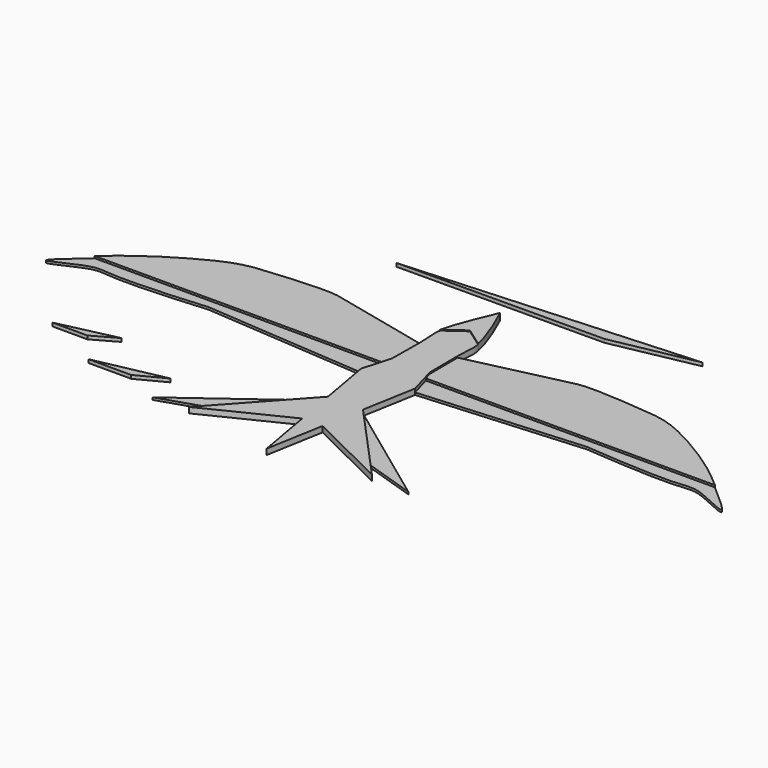
from build123d import *

# Parameters (mm, degrees)
F1_DEPTH = 2
F2_DEPTH = 2.3
F3_DEPTH = 1.5
F4_DEPTH = 0.8
F5_DEPTH = 1.2


# Not quite as in the source:
# - a feature names something its author has since deleted; it is built from what else it names


with BuildPart() as f1:
    # F0 (on Top) → F1 (new body)
    with BuildSketch(Plane.XY):
        with BuildLine():
            Line((-6.6419716499, 2.745028284), (0, 0))
            Line((0, 0), (0, 28.6946911365))
            Line((0, 28.6946911365), (-6.6419716499, 23.9225961235))
            add(Edge.make_bspline(
                [(-6.5175706139, 15.0729201773), (-6.5414876506, 16.2812130784), (-6.6806623081, 20.0881688925), (-7.0635559844, 21.7026716796), (-6.6419716499, 23.9225961235)],
                knots=[0.2785134471, 0.2785134471, 0.2785134471, 0.2785134471, 0.3682433903, 0.5898063865, 0.5898063865, 0.5898063865, 0.5898063865], degree=3))
            add(Edge.make_bspline(
                [(-6.6419716499, 2.745028284), (-6.5251722943, 6.5032297687), (-6.4433343436, 11.3224907311), (-6.5175706139, 15.0729201773)],
                knots=[0, 0, 0, 0, 0.2785134471, 0.2785134471, 0.2785134471, 0.2785134471], degree=3))
        make_face()
        with BuildLine():
            Line((0, 28.6946911365), (0, 0))
            Line((0, 0), (6.6419716499, 2.745028284))
            add(Edge.make_bspline(
                [(6.6419716499, 2.745028284), (6.6625704877, 4.4259580865), (6.6879671442, 8.5489520633), (6.5628964948, 13.2490139748), (6.5686901265, 15.0847156957)],
                knots=[0, 0, 0, 0, 0.2083076988, 0.3619822263, 0.3619822263, 0.3619822263, 0.3619822263], degree=3))
            add(Edge.make_bspline(
                [(6.5686901265, 15.0847156957), (6.5717947616, 16.0684137089), (6.6405692543, 19.2909426976), (7.065262223, 21.4932328604), (6.6419716499, 23.9949107423)],
                knots=[0.3619822263, 0.3619822263, 0.3619822263, 0.3619822263, 0.4443318399, 0.644940685, 0.644940685, 0.644940685, 0.644940685], degree=3))
            Line((6.6419716499, 23.9949107423), (0, 28.6946911365))
        make_face()
        Polygon((9.5007317222, -7.3481148503), (0, -8.0477236517), (0, -38.9328375459), (3.5725845946, -40.6871710497), (6.1658886261, -26.1027980596), align=None)
        Polygon((0, -38.9328375459), (0, -8.0477236517), (-9.5007317222, -7.3481148503), (-6.1658886261, -26.1027980596), (-3.5725845946, -40.6871710497), align=None)
        Polygon((-32.2535888602, -54.7711053479), (-3.5725845946, -40.6871710497), (-6.1658886261, -26.1027980596), (-26.8448407595, -48.8273214495), align=None)
        Polygon((26.8448407595, -48.8273214495), (6.1658886261, -26.1027980596), (3.5725845946, -40.6871710497), (32.2535888602, -54.7711053479), align=None)
        Polygon((0, -8.0477236517), (0, 0), (-7.4194675351, 0), (-9.5007317222, -7.3481148503), align=None)
        Polygon((7.4194675351, 0), (0, 0), (0, -8.0477236517), (9.5007317222, -7.3481148503), align=None)
        Polygon((6.6419716499, 2.745028284), (0, 0), (7.4194675351, 0), align=None)
        Polygon((-7.4194675351, 0), (0, 0), (-6.6419716499, 2.745028284), align=None)
        Polygon((3.5725845946, -40.6871710497), (0, -38.9328375459), (-3.5725845946, -40.6871710497), (0, -60.7788786292), align=None)
    extrude(amount=F1_DEPTH)

    # F0 (on Top) → F3 (join)
    with BuildSketch(Plane.XY):
        with BuildLine():
            Line((6.6419716499, 2.745028284), (7.4194675351, 0))
            Line((7.4194675351, 0), (109.2885956168, 0))
            add(Edge.make_bspline(
                [(42.290057987, 23.3256332576), (46.9602869466, 24.1669337854), (66.2240272129, 22.5460111833), (77.2780101126, 21.5519474786), (97.7039953696, 9.7181396105), (104.4322660293, 4.1460579818), (109.2885956168, 0)],
                knots=[0, 0, 0, 0, 0.1453308986, 0.2550811327, 0.396472964, 0.5191870129, 0.5191870129, 0.5191870129, 0.5191870129], degree=3))
            add(Edge.make_bspline(
                [(42.290057987, 23.3256332576), (30.384955122, 20.5786005266), (18.4738102627, 17.8317479119), (6.5686901266, 15.0847156956)],
                knots=[0, 0, 0, 0, 36.6596267337, 36.6596267337, 36.6596267337, 36.6596267337], degree=3))
            add(Edge.make_bspline(
                [(6.6419716499, 2.745028284), (6.6625704877, 4.4259580865), (6.6879671442, 8.5489520633), (6.5628964948, 13.2490139748), (6.5686901265, 15.0847156957)],
                knots=[0, 0, 0, 0, 0.2083076988, 0.3619822263, 0.3619822263, 0.3619822263, 0.3619822263], degree=3))
        make_face()
        with BuildLine():
            Line((-109.2885956168, 0), (-7.4194675351, 0))
            Line((-7.4194675351, 0), (-6.6419716499, 2.745028284))
            add(Edge.make_bspline(
                [(-6.6419716499, 2.745028284), (-6.5251722943, 6.5032297687), (-6.4433343436, 11.3224907311), (-6.5175706139, 15.0729201773)],
                knots=[0, 0, 0, 0, 0.2785134471, 0.2785134471, 0.2785134471, 0.2785134471], degree=3))
            add(Edge.make_bspline(
                [(-42.290057987, 23.3256332576), (-30.3679152969, 20.5746686867), (-18.4397133041, 17.8238847482), (-6.5175706139, 15.0729201773)],
                knots=[0, 0, 0, 0, 36.7120978158, 36.7120978158, 36.7120978158, 36.7120978158], degree=3))
            add(Edge.make_bspline(
                [(-42.290057987, 23.3256332576), (-46.9602869466, 24.1669337854), (-66.2240272129, 22.5460111833), (-77.2780101126, 21.5519474786), (-97.7039953696, 9.7181396105), (-104.4322660293, 4.1460579818), (-109.2885956168, 0)],
                knots=[0, 0, 0, 0, 0.1453308986, 0.2550811327, 0.396472964, 0.5191870129, 0.5191870129, 0.5191870129, 0.5191870129], degree=3))
        make_face()
    extrude(amount=F3_DEPTH)


with BuildPart() as f2:
    # F0 (on Top) → F2 (new body)
    with BuildSketch(Plane.XY):
        with BuildLine():
            Line((-6.6419716499, 23.9225961235), (0, 28.6946911365))
            Line((0, 28.6946911365), (6.6419716499, 23.9949107423))
            add(Edge.make_bspline(
                [(6.6419716499, 23.9949107423), (5.892786035, 28.4226518758), (2.8744096347, 35.7960231207), (0, 42.0363731682)],
                knots=[0.644940685, 0.644940685, 0.644940685, 0.644940685, 1, 1, 1, 1], degree=3))
            add(Edge.make_bspline(
                [(-6.6419716499, 23.9225961235), (-5.8614658592, 28.032482904), (-2.70186861, 35.812589021), (0, 42.0363731682)],
                knots=[0.5898063865, 0.5898063865, 0.5898063865, 0.5898063865, 1, 1, 1, 1], degree=3))
        make_face()
    extrude(amount=F2_DEPTH)


with BuildPart() as f4:
    # F0 (on Top) → F4 (new body)
    with BuildSketch(Plane.XY):
        with BuildLine():
            Line((-66.6123788172, -3.1425639369), (-109.2885956168, 0))
            add(Edge.make_bspline(
                [(-109.2885956168, 0), (-113.7072309048, -3.7723794842), (-125.0662078985, -13.5985728633), (-106.5027266596, -3.0910792348), (-99.4689310801, -5.3383077024), (-79.0510181663, -4.1965041845), (-66.6123788172, -3.1425639369)],
                knots=[0.5191870129, 0.5191870129, 0.5191870129, 0.5191870129, 0.6308410134, 0.7359516151, 0.8254118404, 1, 1, 1, 1], degree=3))
        make_face()
        Polygon((-9.5007317222, -7.3481148503), (-7.4194675351, 0), (-109.2885956168, 0), (-66.6123788172, -3.1425639369), align=None)
    extrude(amount=F4_DEPTH)


with BuildPart() as f4b:
    # F0 (on Top) → F4, piece 2 (new body)
    with BuildSketch(Plane.XY):
        with BuildLine():
            add(Edge.make_bspline(
                [(109.2885956168, 0), (113.7072309048, -3.7723794842), (125.0662078985, -13.5985728633), (106.5027266596, -3.0910792348), (99.4689310801, -5.3383077024), (79.0510181663, -4.1965041845), (66.6123788172, -3.1425639369)],
                knots=[0.5191870129, 0.5191870129, 0.5191870129, 0.5191870129, 0.6308410134, 0.7359516151, 0.8254118404, 1, 1, 1, 1], degree=3))
            Line((109.2885956168, 0), (66.6123788172, -3.1425639369))
        make_face()
        Polygon((109.2885956168, 0), (7.4194675351, 0), (9.5007317222, -7.3481148503), (66.6123788172, -3.1425639369), align=None)
    extrude(amount=F4_DEPTH)


with BuildPart() as f4c:
    # F0 (on Top) → F4, piece 3 (new body)
    with BuildSketch(Plane.XY):
        Polygon((-26.8448407595, -48.8273214495), (-6.1658886261, -26.1027980596), (-45.1018763415, -54.7711053479), align=None)
    extrude(amount=F4_DEPTH)


with BuildPart() as f4d:
    # F0 (on Top) → F4, piece 4 (new body)
    with BuildSketch(Plane.XY):
        Polygon((45.1018763415, -54.7711053479), (6.1658886261, -26.1027980596), (26.8448407595, -48.8273214495), align=None)
    extrude(amount=F4_DEPTH)


with BuildPart() as f5:
    # F0 (on Top) → F5 (new body)
    with BuildSketch(Plane.XY):
        Polygon((-73.3117833734, -33.1380404532), (-93.9138201779, -37.7803705633), (-81.5899297595, -37.7803705633), align=None)
    extrude(amount=F5_DEPTH)


with BuildPart() as f5b:
    # F0 (on Top) → F5, piece 2 (new body)
    with BuildSketch(Plane.XY):
        Polygon((60.6261715293, 55.3805120289), (-42.1832613647, 49.102075398), (30.8035947382, 49.4944788516), align=None)
    extrude(amount=F5_DEPTH)


with BuildPart() as f5c:
    # F0 (on Top) → F5, piece 3 (new body)
    with BuildSketch(Plane.XY):
        Polygon((-47.6768948138, -43.504897505), (-72.4707837196, -48.6061275005), (-57.4869550765, -48.6061275005), align=None)
    extrude(amount=F5_DEPTH)


solid = Compound([f1.part, f2.part, f4.part, f4b.part, f4c.part, f4d.part, f5.part, f5b.part, f5c.part])
